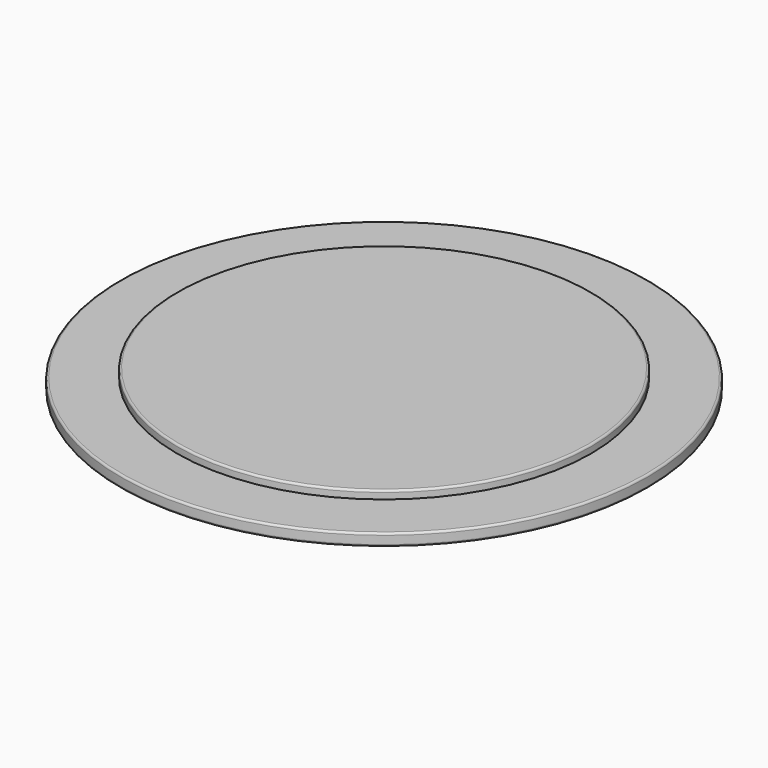
from build123d import *

# Parameters (mm, degrees)
F0_R         = 65
F1_DEPTH     = 3
F2_R         = 51
F3_DEPTH     = 2
F4_R         = 0.5
F5_TEXT_SIZE = 13.8888888889
F6_DEPTH     = 0.5


# Not quite as in the source:
# - Text() gives the source's letters only with a copy of the font that has no kerning and outlines rounded to 1/6400 em; it was checked with that copy


with BuildPart() as f1:
    # F0 (on Top) → F1 (new body)
    with BuildSketch(Plane.XY):
        Circle(F0_R)
    extrude(amount=F1_DEPTH)

    # F2 (on face) → F3 (join)
    with BuildSketch(Plane.XY.offset(3)):
        Circle(F2_R)
    extrude(amount=F3_DEPTH)

    # F4
    f4_edges = [f1.edges().sort_by_distance(p)[0] for p in [
        (65, 0, 1.5),
        (-65, 0, 0),
        (-65, 0, 3),
        (-51, 0, 5),
    ]]
    fillet(f4_edges, radius=F4_R)

    # F5 (on face) → F6 (cut)
    with BuildSketch(Plane(origin=(0, 0, 0), x_dir=(1, 0, 0), z_dir=(0, 0, -1))):
        with Locations((-36.0802651727, 5.3376717638)):
            Text('Sushi  cake', F5_TEXT_SIZE, font='Open Sans', text_align=(TextAlign.LEFT, TextAlign.BOTTOM))
        with Locations((-32.4713242004, -13.5512171251)):
            Text('by DenisG', F5_TEXT_SIZE, font='Open Sans', text_align=(TextAlign.LEFT, TextAlign.BOTTOM))
    extrude(amount=-F6_DEPTH, mode=Mode.SUBTRACT)


solid = f1.part
